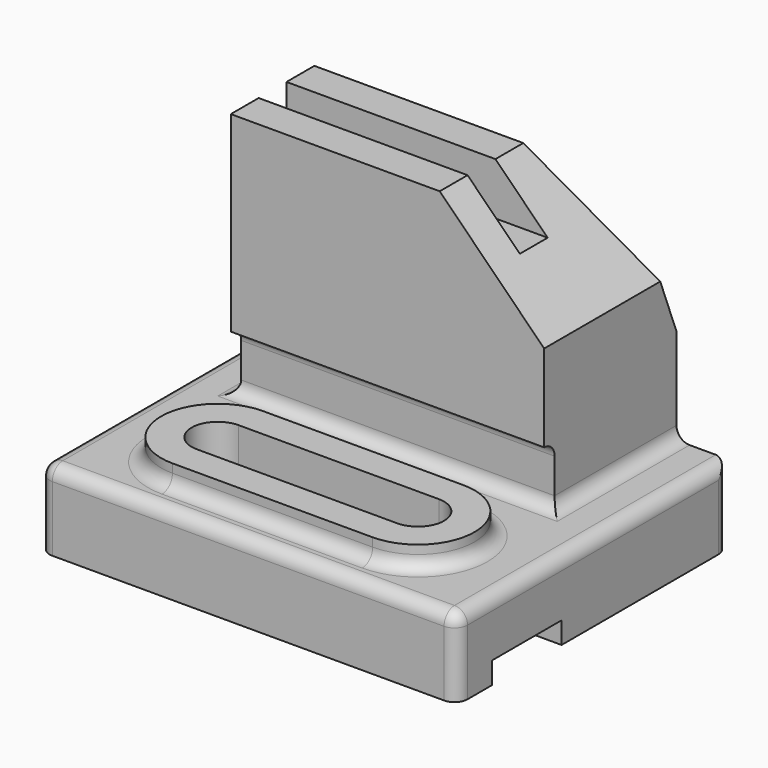
from build123d import *

# Parameters (mm, degrees)
F0_W      = 96
F0_H      = 78
F1_DEPTH  = 18
F2_W      = 72
F2_H      = 38
F4_DEPTH  = 58
F6_DEPTH  = 38
F7_W      = 8
F7_H      = 12
F8_DEPTH  = 60.001
F10_DEPTH = 72.001
F11_W     = 20
F11_H     = 5
F12_DEPTH = 96.001
F13_W     = 46
F13_H     = 26
F14_DEPTH = 5
F17_DEPTH = 23.001
F18_W     = 3
F18_H     = 14
F19_DEPTH = 72
F20_R     = 2.99999


# Not quite as in the source:
# - a fillet or chamfer is up to 0.001 mm smaller than in the source, because OpenCascade refuses the exact size


with BuildPart() as f1:
    # F0 (on Top) → F1 (new body)
    with BuildSketch(Plane.XY):
        with Locations((48, 39)):
            Rectangle(F0_W, F0_H)
    extrude(amount=F1_DEPTH)

    # F2 (on face) → F4 (join, through all)
    with BuildSketch(Plane.XY.offset(18)):
        with Locations((48, 59)):
            Rectangle(F2_W, F2_H)
    extrude(amount=F4_DEPTH)

    # F5 (on face) → F6 (cut, through all)
    with BuildSketch(Plane(origin=(0, 78, 0), x_dir=(-1, 0, 0), z_dir=(0, 1, 0))):
        Polygon((-60, 76), (-84, 76), (-84, 52), align=None)
    extrude(amount=-F6_DEPTH, mode=Mode.SUBTRACT)

    # F7 (on face) → F8 (cut, through all)
    with BuildSketch(Plane(origin=(12, 0, 0), x_dir=(0, -1, 0), z_dir=(-1, 0, 0))):
        with Locations((-52, 70)):
            Rectangle(F7_W, F7_H)
    extrude(amount=-F8_DEPTH, mode=Mode.SUBTRACT)

    # F9 (on face) → F10 (cut, through all)
    with BuildSketch(Plane(origin=(12, 0, 0), x_dir=(0, -1, 0), z_dir=(-1, 0, 0))):
        Polygon((-78, 40), (-64, 76), (-78, 76), align=None)
    extrude(amount=-F10_DEPTH, mode=Mode.SUBTRACT)

    # F11 (on face) → F12 (cut, through all)
    with BuildSketch(Plane.YZ.offset(96)):
        with Locations((20, 2.5)):
            Rectangle(F11_W, F11_H)
    extrude(amount=-F12_DEPTH, mode=Mode.SUBTRACT)

    # F13 (on face) → F14 (join)
    with BuildSketch(Plane.XY.offset(18)):
        with BuildLine():
            Line((25, 7), (25, 33))
            ThreePointArc((25, 33), (12, 20), (25, 7))
        make_face()
        with BuildLine():
            ThreePointArc((71, 7), (84, 20), (71, 33))
            Line((71, 33), (71, 7))
        make_face()
        with Locations((48, 20)):
            Rectangle(F13_W, F13_H)
    extrude(amount=F14_DEPTH)

    # F15 (on face) → F17 (cut, through all)
    with BuildSketch(Plane.XY.offset(23)):
        with BuildLine():
            ThreePointArc((25, 26), (19, 20), (25, 14))
            Line((25, 14), (71, 14))
            ThreePointArc((71, 14), (77, 20), (71, 26))
            Line((71, 26), (25, 26))
        make_face()
    extrude(amount=-F17_DEPTH, mode=Mode.SUBTRACT)

    # F18 (on face) → F19 (cut, through all)
    with BuildSketch(Plane.YZ.offset(84)):
        with Locations((41.5, 25)):
            Rectangle(F18_W, F18_H)
    extrude(amount=-F19_DEPTH, mode=Mode.SUBTRACT)

    # F20 (radius 3 in the source; OpenCascade refuses exactly that, so slightly less here)
    f20_edges = [f1.edges().sort_by_distance(p)[0] for p in [
        (48, 7, 18),
        (48, 43, 18),
        (48, 43, 32),
        (48, 0, 18),
        (0, 39, 18),
        (84, 60.5, 18),
        (12, 60.5, 18),
        (96, 39, 18),
        (96, 0, 9),
        (0, 0, 9),
        (96, 78, 9),
        (0, 78, 9),
    ]]
    fillet(f20_edges, radius=F20_R)


solid = f1.part
